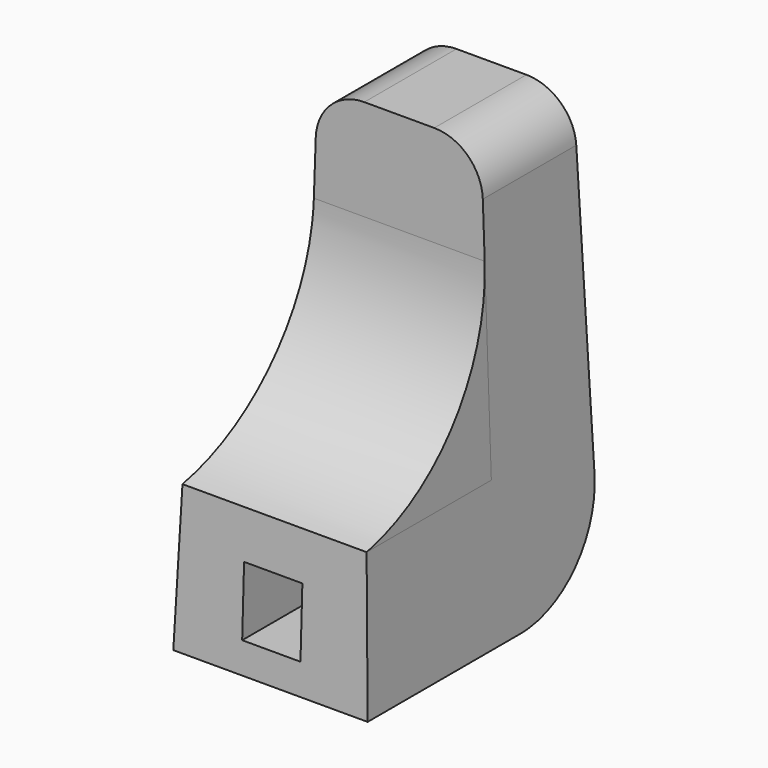
from build123d import *

# Parameters (mm, degrees)
F0_W        = 20
F0_H        = 30
F1_DEPTH    = 45
F1_TAPER    = 2
F4_DEPTH    = 20.001
F5_T4_DEPTH = 116.9802704864
F7_W        = 6
F7_H        = 7
F8_DEPTH    = 10
F9_R        = 5
F10_R       = 10


# Not quite as in the source:
# - a fillet or chamfer that OpenCascade refuses, or shapes differently, is made with other operations: its cross-section is extruded or revolved along the edge and cut away or added


with BuildPart() as f1:
    # F0 (on Top) → F1 (new body)
    with BuildSketch(Plane.XY):
        Rectangle(F0_W, F0_H)
    extrude(amount=F1_DEPTH, taper=F1_TAPER)

    # F3 (on face) → F4 (cut, through all)
    with BuildSketch(Plane(origin=(-10, 0, 0), x_dir=(0, -1, 0), z_dir=(-1, 0, 0))):
        Polygon((14.4761884576, 15), (13.4285653729, 45), (-1.5714346271, 45), (-1.5714346271, 15), (13.4285653729, 15), align=None)
    extrude(amount=-F4_DEPTH, mode=Mode.SUBTRACT)

    # F5: fillet of radius 20 on 1 edges, made by hand


with BuildPart() as f5_tool2:
    # F5_s3 → F5_t4 (new body)
    with BuildSketch(Plane.YZ.offset(-58.4901352432)):
        with BuildLine():
            ThreePointArc((-14.4761884576, 15), (-2.9520099049, 21.9376573833), (1.5714346271, 34.6055787142))
            Line((1.5714346271, 34.6055787142), (1.5714346271, 15))
            Line((1.5714346271, 15), (-14.4761884576, 15))
        make_face()
    extrude(amount=F5_T4_DEPTH)

    split(bisect_by=Plane(origin=(-9.9878202513, 0, 0.3487823687), x_dir=(0, 1, 0), z_dir=(0.999390827, 0, -0.0348994967)), keep=Keep.TOP)

    split(bisect_by=Plane(origin=(9.9878202513, 0, 0.3487823687), x_dir=(0, 1, 0), z_dir=(-0.999390827, 0, -0.0348994967)), keep=Keep.TOP)


with BuildPart() as f1_1:
    add(f1.part)

    # F5_t1: union F5_tool2
    add(f5_tool2.part)

    # F7 (on face) → F8 (cut)
    with BuildSketch(Plane(origin=(0, -15, 0), x_dir=(-1, 0, 0), z_dir=(0, 1, 0))):
        with Locations((0, 6.6315173171)):
            Rectangle(F7_W, F7_H)
    extrude(amount=F8_DEPTH, mode=Mode.SUBTRACT)

    # F9
    f9_edges = [f1_1.edges().sort_by_distance(p)[0] for p in [
        (-8.428565, 7.5, 45),
        (8.428565, 7.5, 45),
    ]]
    fillet(f9_edges, radius=F9_R)

    # F10
    f10_edges = [f1_1.edges().sort_by_distance(p)[0] for p in [
        (0, 15, 0),
    ]]
    fillet(f10_edges, radius=F10_R)


solid = f1_1.part
